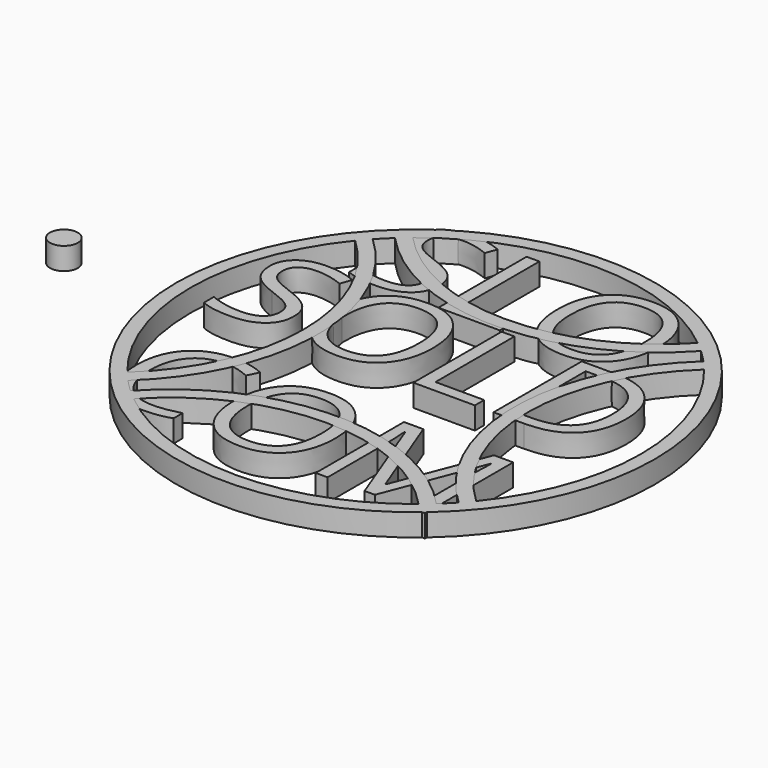
from build123d import *

# Parameters (mm, degrees)
F0_TEXT_SIZE = 27.7777777778
F1_DEPTH     = 4
F2_R         = 43
F3_DEPTH     = 4
F2_R_2       = 2.5


# Not quite as in the source:
# - Text() gives the source's letters only with a copy of the font that has no kerning and outlines rounded to 1/6400 em; it was checked with that copy


with BuildPart() as f1:
    # F0 (on Top) → F1 (new body)
    with BuildSketch(Plane.XY):
        with Locations((-24.6202256944, 10)):
            Text('SOLD', F0_TEXT_SIZE, font='Open Sans', text_align=(TextAlign.LEFT, TextAlign.BOTTOM))
        with Locations((-14.4965277778, 30)):
            Text('SLO', F0_TEXT_SIZE, font='Open Sans', text_align=(TextAlign.LEFT, TextAlign.BOTTOM))
        with Locations((-20.4557291667, -20)):
            Text('COM', F0_TEXT_SIZE, font='Open Sans', text_align=(TextAlign.LEFT, TextAlign.BOTTOM))
    extrude(amount=F1_DEPTH)


with BuildPart() as f3:
    # F2 (on Top) → F3 (new body, through all)
    with BuildSketch(Plane.XY):
        with Locations((13, 13)):
            Circle(F2_R)
        with BuildLine():
            ThreePointArc((44.3728593874, 38.6123738427), (51.1500380419, 26.595021052), (53.5, 13))
            ThreePointArc((53.5, 13), (51.1500380419, -0.595021052), (44.3728593874, -12.6123738427))
            ThreePointArc((44.3728593874, -12.6123738427), (43.5670728745, -13.5688549976), (42.7321374946, -14.5))
            ThreePointArc((42.7321374946, -14.5), (41.6378246381, -15.6378246381), (40.5, -16.7321374946))
            ThreePointArc((40.5, -16.7321374946), (39.5688549976, -17.5670728745), (38.6123738427, -18.3728593874))
            ThreePointArc((38.6123738427, -18.3728593874), (13, -27.5), (-12.6123738427, -18.3728593874))
            ThreePointArc((-12.6123738427, -18.3728593874), (-13.5688549976, -17.5670728745), (-14.5, -16.7321374946))
            ThreePointArc((-14.5, -16.7321374946), (-15.6378246381, -15.6378246381), (-16.7321374946, -14.5))
            ThreePointArc((-16.7321374946, -14.5), (-17.5670728745, -13.5688549976), (-18.3728593874, -12.6123738427))
            ThreePointArc((-18.3728593874, -12.6123738427), (-27.5, 13), (-18.3728593874, 38.6123738427))
            ThreePointArc((-18.3728593874, 38.6123738427), (-17.5670728745, 39.5688549976), (-16.7321374946, 40.5))
            ThreePointArc((-16.7321374946, 40.5), (-15.6378246381, 41.6378246381), (-14.5, 42.7321374946))
            ThreePointArc((-14.5, 42.7321374946), (-13.5688549976, 43.5670728745), (-12.6123738427, 44.3728593874))
            ThreePointArc((-12.6123738427, 44.3728593874), (13, 53.5), (38.6123738427, 44.3728593874))
            ThreePointArc((38.6123738427, 44.3728593874), (39.5688549976, 43.5670728745), (40.5, 42.7321374946))
            ThreePointArc((40.5, 42.7321374946), (41.6378246381, 41.6378246381), (42.7321374946, 40.5))
            ThreePointArc((42.7321374946, 40.5), (43.5670728745, 39.5688549976), (44.3728593874, 38.6123738427))
        make_face(mode=Mode.SUBTRACT)
        with BuildLine():
            ThreePointArc((-16.7321374946, -14.5), (-4.6541183584, 13), (-16.7321374946, 40.5))
            ThreePointArc((-16.7321374946, 40.5), (-17.5670728745, 39.5688549976), (-18.3728593874, 38.6123738427))
            ThreePointArc((-18.3728593874, 38.6123738427), (-7.1541183584, 13), (-18.3728593874, -12.6123738427))
            ThreePointArc((-18.3728593874, -12.6123738427), (-17.5670728745, -13.5688549976), (-16.7321374946, -14.5))
        make_face()
        with BuildLine():
            ThreePointArc((-14.5, 42.7321374946), (13, 30.6541183584), (40.5, 42.7321374946))
            ThreePointArc((40.5, 42.7321374946), (39.5688549976, 43.5670728745), (38.6123738427, 44.3728593874))
            ThreePointArc((38.6123738427, 44.3728593874), (13, 33.1541183584), (-12.6123738427, 44.3728593874))
            ThreePointArc((-12.6123738427, 44.3728593874), (-13.5688549976, 43.5670728745), (-14.5, 42.7321374946))
        make_face()
        with BuildLine():
            ThreePointArc((44.3728593874, -12.6123738427), (33.1541183584, 13), (44.3728593874, 38.6123738427))
            ThreePointArc((44.3728593874, 38.6123738427), (43.5670728745, 39.5688549976), (42.7321374946, 40.5))
            ThreePointArc((42.7321374946, 40.5), (30.6541183584, 13), (42.7321374946, -14.5))
            ThreePointArc((42.7321374946, -14.5), (43.5670728745, -13.5688549976), (44.3728593874, -12.6123738427))
        make_face()
        with BuildLine():
            ThreePointArc((38.6123738427, -18.3728593874), (39.5688549976, -17.5670728745), (40.5, -16.7321374946))
            ThreePointArc((40.5, -16.7321374946), (13, -4.6541183584), (-14.5, -16.7321374946))
            ThreePointArc((-14.5, -16.7321374946), (-13.5688549976, -17.5670728745), (-12.6123738427, -18.3728593874))
            ThreePointArc((-12.6123738427, -18.3728593874), (13, -7.1541183584), (38.6123738427, -18.3728593874))
        make_face()
    extrude(amount=F3_DEPTH)


with BuildPart() as f3b:
    # F2 (on Top) → F3, piece 2 (new body, through all)
    with BuildSketch(Plane.XY):
        with Locations((-50.8750788867, 13.7686338276)):
            Circle(F2_R_2)
    extrude(amount=F3_DEPTH)


solid = Compound([f1.part, f3.part, f3b.part])
